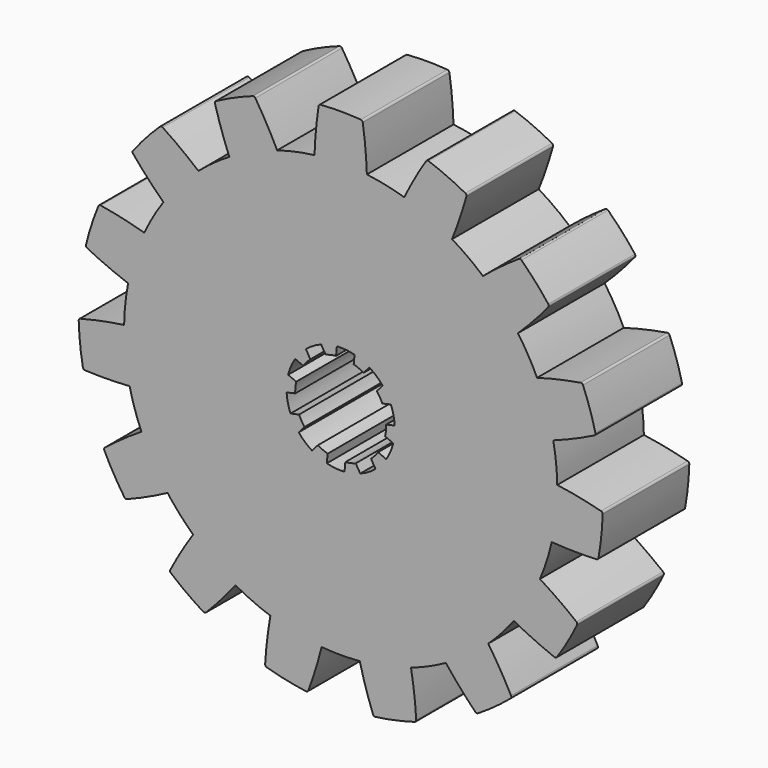
from build123d import *

# Parameters (mm, degrees)
F1_DEPTH = 25
F2_R     = 0.5


with BuildPart() as f1:
    # F0 (on Front) → F1 (new body)
    with BuildSketch(Plane.XZ):
        with BuildLine():
            ThreePointArc((10.4971477332, 0.2447232447), (10.4992869091, 0.1223699329), (10.5, 0))
            ThreePointArc((10.5, 0), (10.4410612014, -1.1109639904), (10.2649064785, -2.2094558126))
            Line((10.2649064785, -2.2094558126), (12.1304516775, -3.0169756546))
            ThreePointArc((12.1304516775, -3.0169756546), (11.6166464297, -4.6155742575), (10.8932201298, -6.1308853524))
            ThreePointArc((10.8932201298, -6.1308853524), (23.5477437836, -20.2652991426), (38.8839835977, -31.433037072))
            ThreePointArc((38.8839835977, -31.433037072), (39.4284740968, -30.7472833011), (39.9608722277, -30.0520996073))
            ThreePointArc((39.9608722277, -30.0520996073), (24.8392901888, -19.9261256688), (12.0639319684, -6.9651143695))
            ThreePointArc((12.0639319684, -6.9651143695), (29.6761761226, -11.5483934811), (46.0063178108, -19.5810807029))
            ThreePointArc((46.0063178108, -19.5810807029), (47.5528258148, -15.4508497187), (48.7293634187, -11.2004080646))
            ThreePointArc((48.7293634187, -11.2004080646), (30.7965061871, -8.1003720854), (13.8539174883, -1.456105403))
            ThreePointArc((13.8539174883, -1.456105403), (31.8076906944, 1.5204058477), (49.9932056918, 0.8242479348))
            ThreePointArc((49.9932056918, 0.8242479348), (49.7260947684, 5.2264231634), (49.0721049822, 9.587935785))
            ThreePointArc((49.0721049822, 9.587935785), (31.4287264881, 5.1260094212), (13.2484348156, 4.3046774159))
            ThreePointArc((13.2484348156, 4.3046774159), (28.4393665814, 14.326313193), (45.3358141347, 21.0870566164))
            ThreePointArc((45.3358141347, 21.0870566164), (43.3012701892, 25), (40.9298337882, 28.7184384337))
            ThreePointArc((40.9298337882, 28.7184384337), (26.6266344584, 17.4660573305), (10.352177405, 9.3211424028))
            ThreePointArc((10.352177405, 9.3211424028), (20.1536176229, 24.6550708367), (32.8394484508, 37.7037216393))
            ThreePointArc((32.8394484508, 37.7037216393), (29.3892626146, 40.4508497187), (25.7104224964, 42.8832621783))
            ThreePointArc((25.7104224964, 42.8832621783), (17.2205554354, 26.7860652532), (5.6659344745, 12.7258971883))
            ThreePointArc((5.6659344745, 12.7258971883), (8.3831250875, 30.7207427485), (14.6648437927, 47.8010706631))
            ThreePointArc((14.6648437927, 47.8010706631), (10.3955845409, 48.9073800367), (6.0454455831, 49.6331803102))
            ThreePointArc((6.0454455831, 49.6331803102), (4.8368859338, 31.4745191499), (0, 13.9302287389))
            ThreePointArc((0, 13.9302287389), (-4.8368859338, 31.4745191499), (-6.0454455831, 49.6331803102))
            ThreePointArc((-6.0454455831, 49.6331803102), (-10.3955845409, 48.9073800367), (-14.6648437927, 47.8010706631))
            ThreePointArc((-14.6648437927, 47.8010706631), (-8.3831250875, 30.7207427485), (-5.6659344745, 12.7258971883))
            ThreePointArc((-5.6659344745, 12.7258971883), (-17.2205554354, 26.7860652532), (-25.7104224964, 42.8832621783))
            ThreePointArc((-25.7104224964, 42.8832621783), (-29.3892626146, 40.4508497187), (-32.8394484508, 37.7037216393))
            ThreePointArc((-32.8394484508, 37.7037216393), (-20.1536176229, 24.6550708367), (-10.352177405, 9.3211424028))
            ThreePointArc((-10.352177405, 9.3211424028), (-26.6266344584, 17.4660573305), (-40.9298337882, 28.7184384337))
            ThreePointArc((-40.9298337882, 28.7184384337), (-43.3012701892, 25), (-45.3358141347, 21.0870566164))
            ThreePointArc((-45.3358141347, 21.0870566164), (-28.4393665814, 14.326313193), (-13.2484348156, 4.3046774159))
            ThreePointArc((-13.2484348156, 4.3046774159), (-31.4287264881, 5.1260094212), (-49.0721049822, 9.587935785))
            ThreePointArc((-49.0721049822, 9.587935785), (-49.7260947684, 5.2264231634), (-49.9932056918, 0.8242479348))
            ThreePointArc((-49.9932056918, 0.8242479348), (-31.8076906944, 1.5204058477), (-13.8539174883, -1.456105403))
            ThreePointArc((-13.8539174883, -1.456105403), (-30.7965061871, -8.1003720854), (-48.7293634187, -11.2004080646))
            ThreePointArc((-48.7293634187, -11.2004080646), (-47.5528258148, -15.4508497187), (-46.0063178108, -19.5810807029))
            ThreePointArc((-46.0063178108, -19.5810807029), (-29.6761761226, -11.5483934811), (-12.0639319684, -6.9651143695))
            ThreePointArc((-12.0639319684, -6.9651143695), (-24.8392901888, -19.9261256688), (-39.9608722277, -30.0520996073))
            ThreePointArc((-39.9608722277, -30.0520996073), (-39.4284740968, -30.7472833011), (-38.8839835977, -31.433037072))
            ThreePointArc((-38.8839835977, -31.433037072), (-22.7114177897, -19.4996773256), (-9.5904018131, -4.2748325187))
            ThreePointArc((-9.5904018131, -4.2748325187), (-9.5967963441, -4.2604577137), (-9.603169329, -4.2460733435))
            Line((-9.603169329, -4.2460733435), (-11.5870753528, -4.6893160234))
            ThreePointArc((-11.5870753528, -4.6893160234), (-12.199238106, -2.7255439153), (-12.4810537571, -0.6879659247))
            Line((-12.4810537571, -0.6879659247), (-10.4971477332, -0.2447232447))
            ThreePointArc((-10.4971477332, -0.2447232447), (-10.4532995979, 0.9892054973), (-10.2649064785, 2.2094558126))
            Line((-10.2649064785, 2.2094558126), (-12.1304516775, 3.0169756546))
            ThreePointArc((-12.1304516775, 3.0169756546), (-11.471425464, 4.9655209015), (-10.5017608218, 6.7796032068))
            Line((-10.5017608218, 6.7796032068), (-8.6362156228, 5.9720833648))
            ThreePointArc((-8.6362156228, 5.9720833648), (-7.8754566192, 6.9445793997), (-7.0057982445, 7.821047945))
            Line((-7.0057982445, 7.821047945), (-8.0404077602, 9.5708851759))
            ThreePointArc((-8.0404077602, 9.5708851759), (-6.3619181943, 10.7599255058), (-4.5111521943, 11.6575943436))
            Line((-4.5111521943, 11.6575943436), (-3.4765426786, 9.9077571127))
            ThreePointArc((-3.4765426786, 9.9077571127), (-2.2894568889, 10.247360009), (-1.0707131994, 10.4452655899))
            Line((-1.0707131994, 10.4452655899), (-0.8792013619, 12.4690418624))
            ThreePointArc((-0.8792013619, 12.4690418624), (1.1776255921, 12.4444042832), (3.202563243, 12.0827806682))
            Line((3.202563243, 12.0827806682), (3.0110514055, 10.0590043957))
            ThreePointArc((3.0110514055, 10.0590043957), (4.1710375573, 9.6359973898), (5.2733478956, 9.0797468011))
            Line((5.2733478956, 9.0797468011), (6.6178300736, 10.6044483646))
            ThreePointArc((6.6178300736, 10.6044483646), (8.2673564283, 9.3755435943), (9.6930083726, 7.8927554561))
            Line((9.6930083726, 7.8927554561), (8.3485261945, 6.3680538926))
            ThreePointArc((8.3485261945, 6.3680538926), (9.0383374248, 5.3440112832), (9.603169329, 4.2460733435))
            Line((9.603169329, 4.2460733435), (11.5870753528, 4.6893160234))
            ThreePointArc((11.5870753528, 4.6893160234), (12.199238106, 2.7255439153), (12.4810537571, 0.6879659247))
            Line((12.4810537571, 0.6879659247), (10.4971477332, 0.2447232447))
        make_face()
        with BuildLine():
            Line((10.5017608218, -6.7796032068), (8.6362156228, -5.9720833648))
            ThreePointArc((8.6362156228, -5.9720833648), (7.8754566192, -6.9445793997), (7.0057982445, -7.821047945))
            Line((7.0057982445, -7.821047945), (8.0404077602, -9.5708851759))
            ThreePointArc((8.0404077602, -9.5708851759), (6.3619181943, -10.7599255058), (4.5111521943, -11.6575943436))
            Line((4.5111521943, -11.6575943436), (3.4765426786, -9.9077571127))
            ThreePointArc((3.4765426786, -9.9077571127), (2.2894568889, -10.247360009), (1.0707131994, -10.4452655899))
            Line((1.0707131994, -10.4452655899), (0.8792013619, -12.4690418624))
            ThreePointArc((0.8792013619, -12.4690418624), (-1.1776255921, -12.4444042832), (-3.202563243, -12.0827806682))
            Line((-3.202563243, -12.0827806682), (-3.0110514055, -10.0590043957))
            ThreePointArc((-3.0110514055, -10.0590043957), (-4.1710375573, -9.6359973898), (-5.2733478956, -9.0797468011))
            Line((-5.2733478956, -9.0797468011), (-6.6178300736, -10.6044483646))
            ThreePointArc((-6.6178300736, -10.6044483646), (-8.2673564283, -9.3755435943), (-9.6930083726, -7.8927554561))
            Line((-9.6930083726, -7.8927554561), (-8.3485261945, -6.3680538926))
            ThreePointArc((-8.3485261945, -6.3680538926), (-9.0303199526, -5.3575480916), (-9.5904018131, -4.2748325187))
            ThreePointArc((-9.5904018131, -4.2748325187), (-22.7114177897, -19.4996773256), (-38.8839835977, -31.433037072))
            ThreePointArc((-38.8839835977, -31.433037072), (-36.5656549106, -34.1020949644), (-34.064519626, -36.6006625985))
            ThreePointArc((-34.064519626, -36.6006625985), (-22.4133810996, -22.6203706631), (-8.1879830138, -11.2697917853))
            ThreePointArc((-8.1879830138, -11.2697917853), (-14.587135259, -28.3064711009), (-24.2827831954, -43.7075101131))
            ThreePointArc((-24.2827831954, -43.7075101131), (-20.3368321538, -45.6772728821), (-16.2326565314, -47.2916574242))
            ThreePointArc((-16.2326565314, -47.2916574242), (-11.2751088653, -29.7810802579), (-2.8962574106, -13.6258198186))
            ThreePointArc((-2.8962574106, -13.6258198186), (-1.812732123, -31.7923705235), (-4.4059803465, -49.8054950501))
            ThreePointArc((-4.4059803465, -49.8054950501), (0, -50), (4.4059803465, -49.8054950501))
            ThreePointArc((4.4059803465, -49.8054950501), (1.812732123, -31.7923705235), (2.8962574106, -13.6258198186))
            ThreePointArc((2.8962574106, -13.6258198186), (11.2751088653, -29.7810802579), (16.2326565314, -47.2916574242))
            ThreePointArc((16.2326565314, -47.2916574242), (20.3368321538, -45.6772728821), (24.2827831954, -43.7075101131))
            ThreePointArc((24.2827831954, -43.7075101131), (14.587135259, -28.3064711009), (8.1879830138, -11.2697917853))
            ThreePointArc((8.1879830138, -11.2697917853), (22.4133810996, -22.6203706631), (34.064519626, -36.6006625985))
            ThreePointArc((34.064519626, -36.6006625985), (36.5656549106, -34.1020949644), (38.8839835977, -31.433037072))
            ThreePointArc((38.8839835977, -31.433037072), (23.5477437836, -20.2652991426), (10.8932201298, -6.1308853524))
            ThreePointArc((10.8932201298, -6.1308853524), (10.7024067944, -6.4582109603), (10.5017608218, -6.7796032068))
        make_face()
        with BuildLine():
            ThreePointArc((39.5127690163, -45.8147474582), (36.9257526611, -41.1266334471), (34.064519626, -36.6006625985))
            ThreePointArc((34.064519626, -36.6006625985), (29.3892626146, -40.4508497187), (24.2827831954, -43.7075101131))
            ThreePointArc((24.2827831954, -43.7075101131), (27.7030676308, -47.827306344), (31.3622969917, -51.7364120075))
            ThreePointArc((31.3622969917, -51.7364120075), (35.5610077637, -48.9455281597), (39.5127690163, -45.8147474582))
        make_face()
        with BuildLine():
            ThreePointArc((24.2827831954, -43.7075101131), (29.3892626146, -40.4508497187), (34.064519626, -36.6006625985))
            ThreePointArc((34.064519626, -36.6006625985), (22.4133810996, -22.6203706631), (8.1879830138, -11.2697917853))
            ThreePointArc((8.1879830138, -11.2697917853), (14.587135259, -28.3064711009), (24.2827831954, -43.7075101131))
        make_face()
        with BuildLine():
            ThreePointArc((12.0639319684, -6.9651143695), (24.8392901888, -19.9261256688), (39.9608722277, -30.0520996073))
            ThreePointArc((39.9608722277, -30.0520996073), (43.3012701892, -25), (46.0063178108, -19.5810807029))
            ThreePointArc((46.0063178108, -19.5810807029), (29.6761761226, -11.5483934811), (12.0639319684, -6.9651143695))
        make_face()
        with BuildLine():
            ThreePointArc((46.0063178108, -19.5810807029), (43.3012701892, -25), (39.9608722277, -30.0520996073))
            ThreePointArc((39.9608722277, -30.0520996073), (44.7611296266, -32.4245657308), (49.6939785027, -34.5073687866))
            ThreePointArc((49.6939785027, -34.5073687866), (52.394536929, -30.25), (54.7312472383, -25.7825634052))
            ThreePointArc((54.7312472383, -25.7825634052), (50.4610624428, -22.5519924933), (46.0063178108, -19.5810807029))
        make_face()
        with BuildLine():
            ThreePointArc((17.4621740692, -57.9251454618), (17.0056447843, -52.5901058542), (16.2326565314, -47.2916574242))
            ThreePointArc((16.2326565314, -47.2916574242), (10.3955845409, -48.9073800367), (4.4059803465, -49.8054950501))
            ThreePointArc((4.4059803465, -49.8054950501), (5.8548935672, -54.9602711929), (7.6077894133, -60.0197595817))
            ThreePointArc((7.6077894133, -60.0197595817), (12.5786572945, -59.1779298444), (17.4621740692, -57.9251454618))
        make_face()
        with BuildLine():
            ThreePointArc((4.4059803465, -49.8054950501), (10.3955845409, -48.9073800367), (16.2326565314, -47.2916574242))
            ThreePointArc((16.2326565314, -47.2916574242), (11.2751088653, -29.7810802579), (2.8962574106, -13.6258198186))
            ThreePointArc((2.8962574106, -13.6258198186), (1.812732123, -31.7923705235), (4.4059803465, -49.8054950501))
        make_face()
        with BuildLine():
            ThreePointArc((13.8539174883, -1.456105403), (30.7965061871, -8.1003720854), (48.7293634187, -11.2004080646))
            ThreePointArc((48.7293634187, -11.2004080646), (49.6813253191, -5.6361258444), (50, 0))
            ThreePointArc((50, 0), (49.9983013941, 0.4121379686), (49.9932056918, 0.8242479348))
            ThreePointArc((49.9932056918, 0.8242479348), (31.8076906944, 1.5204058477), (13.8539174883, -1.456105403))
        make_face()
        with BuildLine():
            ThreePointArc((50, 0), (49.6813253191, -5.6361258444), (48.7293634187, -11.2004080646))
            ThreePointArc((48.7293634187, -11.2004080646), (54.0795856679, -11.4153231348), (59.433119675, -11.3116880129))
            ThreePointArc((59.433119675, -11.3116880129), (60.1685746698, -6.3239720277), (60.486195595, -1.2923399121))
            ThreePointArc((60.486195595, -1.2923399121), (55.2711961039, -0.077907159), (49.9932056918, 0.8242479348))
            ThreePointArc((49.9932056918, 0.8242479348), (49.9983013941, 0.4121379686), (50, 0))
        make_face()
        with BuildLine():
            ThreePointArc((-7.6077894133, -60.0197595817), (-5.8548935672, -54.9602711929), (-4.4059803465, -49.8054950501))
            ThreePointArc((-4.4059803465, -49.8054950501), (-10.3955845409, -48.9073800367), (-16.2326565314, -47.2916574242))
            ThreePointArc((-16.2326565314, -47.2916574242), (-17.0056447843, -52.5901058542), (-17.4621740692, -57.9251454618))
            ThreePointArc((-17.4621740692, -57.9251454618), (-12.5786572945, -59.1779298444), (-7.6077894133, -60.0197595817))
        make_face()
        with BuildLine():
            ThreePointArc((-16.2326565314, -47.2916574242), (-10.3955845409, -48.9073800367), (-4.4059803465, -49.8054950501))
            ThreePointArc((-4.4059803465, -49.8054950501), (-1.812732123, -31.7923705235), (-2.8962574106, -13.6258198186))
            ThreePointArc((-2.8962574106, -13.6258198186), (-11.2751088653, -29.7810802579), (-16.2326565314, -47.2916574242))
        make_face()
        with BuildLine():
            ThreePointArc((13.2484348156, 4.3046774159), (31.4287264881, 5.1260094212), (49.0721049822, 9.587935785))
            ThreePointArc((49.0721049822, 9.587935785), (47.5528258148, 15.4508497187), (45.3358141347, 21.0870566164))
            ThreePointArc((45.3358141347, 21.0870566164), (28.4393665814, 14.326313193), (13.2484348156, 4.3046774159))
        make_face()
        with BuildLine():
            ThreePointArc((45.3358141347, 21.0870566164), (47.5528258148, 15.4508497187), (49.0721049822, 9.587935785))
            ThreePointArc((49.0721049822, 9.587935785), (54.0471900496, 11.5677325362), (58.8957345225, 13.8398863816))
            ThreePointArc((58.8957345225, 13.8398863816), (57.5389192359, 18.6955281597), (55.7825312334, 23.4213408923))
            ThreePointArc((55.7825312334, 23.4213408923), (50.5244378355, 22.4096490308), (45.3358141347, 21.0870566164))
        make_face()
        with BuildLine():
            ThreePointArc((-31.3622969917, -51.7364120075), (-27.7030676308, -47.827306344), (-24.2827831954, -43.7075101131))
            ThreePointArc((-24.2827831954, -43.7075101131), (-29.3892626146, -40.4508497187), (-34.064519626, -36.6006625985))
            ThreePointArc((-34.064519626, -36.6006625985), (-36.9257526611, -41.1266334471), (-39.5127690164, -45.8147474582))
            ThreePointArc((-39.5127690164, -45.8147474582), (-35.5610077637, -48.9455281597), (-31.3622969917, -51.7364120075))
        make_face()
        with BuildLine():
            ThreePointArc((-34.064519626, -36.6006625985), (-29.3892626146, -40.4508497187), (-24.2827831954, -43.7075101131))
            ThreePointArc((-24.2827831954, -43.7075101131), (-14.587135259, -28.3064711009), (-8.1879830138, -11.2697917853))
            ThreePointArc((-8.1879830138, -11.2697917853), (-22.4133810996, -22.6203706631), (-34.064519626, -36.6006625985))
        make_face()
        with BuildLine():
            ThreePointArc((-49.6939785027, -34.5073687866), (-44.7611296266, -32.4245657308), (-39.9608722277, -30.0520996073))
            ThreePointArc((-39.9608722277, -30.0520996073), (-43.3012701892, -25), (-46.0063178108, -19.5810807029))
            ThreePointArc((-46.0063178108, -19.5810807029), (-50.4610624428, -22.5519924933), (-54.7312472383, -25.7825634052))
            ThreePointArc((-54.7312472383, -25.7825634052), (-52.394536929, -30.25), (-49.6939785027, -34.5073687866))
        make_face()
        with BuildLine():
            ThreePointArc((-46.0063178108, -19.5810807029), (-43.3012701892, -25), (-39.9608722277, -30.0520996073))
            ThreePointArc((-39.9608722277, -30.0520996073), (-24.8392901888, -19.9261256688), (-12.0639319684, -6.9651143695))
            ThreePointArc((-12.0639319684, -6.9651143695), (-29.6761761226, -11.5483934811), (-46.0063178108, -19.5810807029))
        make_face()
        with BuildLine():
            ThreePointArc((10.352177405, 9.3211424028), (26.6266344584, 17.4660573305), (40.9298337882, 28.7184384337))
            ThreePointArc((40.9298337882, 28.7184384337), (37.1572412739, 33.4565303179), (32.8394484508, 37.7037216393))
            ThreePointArc((32.8394484508, 37.7037216393), (20.1536176229, 24.6550708367), (10.352177405, 9.3211424028))
        make_face()
        with BuildLine():
            ThreePointArc((32.8394484508, 37.7037216393), (37.1572412739, 33.4565303179), (40.9298337882, 28.7184384337))
            ThreePointArc((40.9298337882, 28.7184384337), (44.6695442683, 32.5506221621), (48.1747418201, 36.5984186894))
            ThreePointArc((48.1747418201, 36.5984186894), (44.9602619414, 40.4824016847), (41.4335604532, 44.0852590802))
            ThreePointArc((41.4335604532, 44.0852590802), (37.0415452653, 41.022373318), (32.8394484508, 37.7037216393))
        make_face()
        with BuildLine():
            ThreePointArc((-59.433119675, -11.3116880129), (-54.0795856679, -11.4153231348), (-48.7293634187, -11.2004080646))
            ThreePointArc((-48.7293634187, -11.2004080646), (-49.7260947684, -5.2264231634), (-49.9932056918, 0.8242479348))
            ThreePointArc((-49.9932056918, 0.8242479348), (-55.2711961039, -0.077907159), (-60.486195595, -1.2923399121))
            ThreePointArc((-60.486195595, -1.2923399121), (-60.1685746698, -6.3239720277), (-59.433119675, -11.3116880129))
        make_face()
        with BuildLine():
            ThreePointArc((-49.9932056918, 0.8242479348), (-49.7260947684, -5.2264231634), (-48.7293634187, -11.2004080646))
            ThreePointArc((-48.7293634187, -11.2004080646), (-30.7965061871, -8.1003720854), (-13.8539174883, -1.456105403))
            ThreePointArc((-13.8539174883, -1.456105403), (-31.8076906944, 1.5204058477), (-49.9932056918, 0.8242479348))
        make_face()
        with BuildLine():
            ThreePointArc((5.6659344745, 12.7258971883), (17.2205554354, 26.7860652532), (25.7104224964, 42.8832621783))
            ThreePointArc((25.7104224964, 42.8832621783), (20.3368321538, 45.6772728821), (14.6648437927, 47.8010706631))
            ThreePointArc((14.6648437927, 47.8010706631), (8.3831250875, 30.7207427485), (5.6659344745, 12.7258971883))
        make_face()
        with BuildLine():
            ThreePointArc((14.6648437927, 47.8010706631), (20.3368321538, 45.6772728821), (25.7104224964, 42.8832621783))
            ThreePointArc((25.7104224964, 42.8832621783), (27.5681284731, 47.905213503), (29.1238986033, 53.0287519196))
            ThreePointArc((29.1238986033, 53.0287519196), (24.6075669061, 55.2695001874), (19.9203506586, 57.1264354711))
            ThreePointArc((19.9203506586, 57.1264354711), (17.1538330068, 52.5419565819), (14.6648437927, 47.8010706631))
        make_face()
        with BuildLine():
            ThreePointArc((-58.8957345225, 13.8398863816), (-54.0471900496, 11.5677325362), (-49.0721049822, 9.587935785))
            ThreePointArc((-49.0721049822, 9.587935785), (-47.5528258148, 15.4508497187), (-45.3358141347, 21.0870566164))
            ThreePointArc((-45.3358141347, 21.0870566164), (-50.5244378355, 22.4096490308), (-55.7825312334, 23.4213408923))
            ThreePointArc((-55.7825312334, 23.4213408923), (-57.5389192359, 18.6955281597), (-58.8957345225, 13.8398863816))
        make_face()
        with BuildLine():
            ThreePointArc((-45.3358141347, 21.0870566164), (-47.5528258148, 15.4508497187), (-49.0721049822, 9.587935785))
            ThreePointArc((-49.0721049822, 9.587935785), (-31.4287264881, 5.1260094212), (-13.2484348156, 4.3046774159))
            ThreePointArc((-13.2484348156, 4.3046774159), (-28.4393665814, 14.326313193), (-45.3358141347, 21.0870566164))
        make_face()
        with BuildLine():
            ThreePointArc((0, 13.9302287389), (4.8368859338, 31.4745191499), (6.0454455831, 49.6331803102))
            ThreePointArc((6.0454455831, 49.6331803102), (0, 50), (-6.0454455831, 49.6331803102))
            ThreePointArc((-6.0454455831, 49.6331803102), (-4.8368859338, 31.4745191499), (0, 13.9302287389))
        make_face()
        with BuildLine():
            ThreePointArc((-6.0454455831, 49.6331803102), (0, 50), (6.0454455831, 49.6331803102))
            ThreePointArc((6.0454455831, 49.6331803102), (5.6999328162, 54.9765582241), (5.0372687356, 60.2899321917))
            ThreePointArc((5.0372687356, 60.2899321917), (0, 60.5), (-5.0372687356, 60.2899321917))
            ThreePointArc((-5.0372687356, 60.2899321917), (-5.6999328162, 54.9765582241), (-6.0454455831, 49.6331803102))
        make_face()
        with BuildLine():
            ThreePointArc((-48.1747418201, 36.5984186894), (-44.6695442683, 32.5506221621), (-40.9298337882, 28.7184384337))
            ThreePointArc((-40.9298337882, 28.7184384337), (-37.1572412739, 33.4565303179), (-32.8394484508, 37.7037216393))
            ThreePointArc((-32.8394484508, 37.7037216393), (-37.0415452653, 41.022373318), (-41.4335604532, 44.0852590802))
            ThreePointArc((-41.4335604532, 44.0852590802), (-44.9602619414, 40.4824016847), (-48.1747418201, 36.5984186894))
        make_face()
        with BuildLine():
            ThreePointArc((-32.8394484508, 37.7037216393), (-37.1572412739, 33.4565303179), (-40.9298337882, 28.7184384337))
            ThreePointArc((-40.9298337882, 28.7184384337), (-26.6266344584, 17.4660573305), (-10.352177405, 9.3211424028))
            ThreePointArc((-10.352177405, 9.3211424028), (-20.1536176229, 24.6550708367), (-32.8394484508, 37.7037216393))
        make_face()
        with BuildLine():
            ThreePointArc((-5.6659344745, 12.7258971883), (-8.3831250875, 30.7207427485), (-14.6648437927, 47.8010706631))
            ThreePointArc((-14.6648437927, 47.8010706631), (-20.3368321538, 45.6772728821), (-25.7104224964, 42.8832621783))
            ThreePointArc((-25.7104224964, 42.8832621783), (-17.2205554354, 26.7860652532), (-5.6659344745, 12.7258971883))
        make_face()
        with BuildLine():
            ThreePointArc((-25.7104224964, 42.8832621783), (-20.3368321538, 45.6772728821), (-14.6648437927, 47.8010706631))
            ThreePointArc((-14.6648437927, 47.8010706631), (-17.1538330068, 52.5419565819), (-19.9203506586, 57.1264354711))
            ThreePointArc((-19.9203506586, 57.1264354711), (-24.6075669061, 55.2695001874), (-29.1238986033, 53.0287519196))
            ThreePointArc((-29.1238986033, 53.0287519196), (-27.5681284731, 47.905213503), (-25.7104224964, 42.8832621783))
        make_face()
    extrude(amount=F1_DEPTH)

    # F2
    f2_edges = [f1.edges().sort_by_distance(p)[0] for p in [
        (-5.037269, -12.5, 60.289932),
        (19.920351, -12.5, 57.126435),
        (29.123899, -12.5, 53.028752),
        (41.43356, -12.5, 44.085259),
        (48.174742, -12.5, 36.598419),
        (55.782531, -12.5, 23.421341),
        (58.895735, -12.5, 13.839886),
        (-19.920351, -12.5, 57.126435),
        (-29.123899, -12.5, 53.028752),
        (-41.43356, -12.5, 44.085259),
        (-48.174742, -12.5, 36.598419),
        (-55.782531, -12.5, 23.421341),
        (-58.895735, -12.5, 13.839886),
        (-60.486196, -12.5, -1.29234),
        (-59.43312, -12.5, -11.311688),
        (-54.731247, -12.5, -25.782563),
        (-49.693979, -12.5, -34.507369),
        (-39.512769, -12.5, -45.814747),
        (-31.362297, -12.5, -51.736412),
        (-17.462174, -12.5, -57.925145),
        (-7.607789, -12.5, -60.01976),
        (7.607789, -12.5, -60.01976),
        (17.462174, -12.5, -57.925145),
        (31.362297, -12.5, -51.736412),
        (39.512769, -12.5, -45.814747),
        (49.693979, -12.5, -34.507369),
        (54.731247, -12.5, -25.782563),
        (59.43312, -12.5, -11.311688),
        (60.486196, -12.5, -1.29234),
        (5.037269, -12.5, 60.289932),
    ]]
    fillet(f2_edges, radius=F2_R)


solid = f1.part
